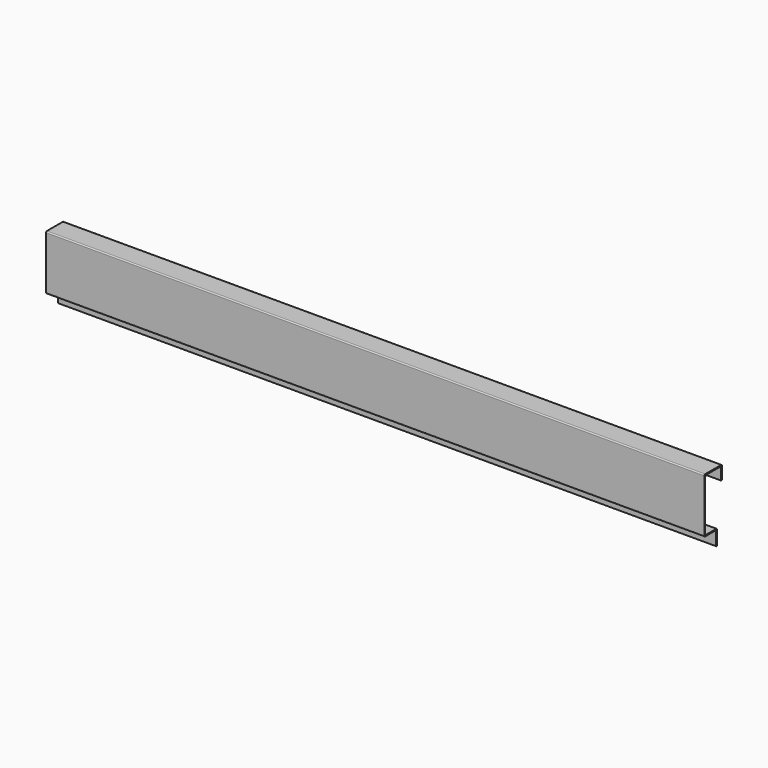
from build123d import *

# Parameters (mm, degrees)
F1_DEPTH = 1200
F3_D     = 5
F4_R     = 2


# Not quite as in the source:
# - a feature names something its author has since deleted; it is built from what else it names


with BuildPart() as f1:
    # F0 (on Right) → F1 (new body)
    with BuildSketch(Plane.YZ):
        Polygon((-18.8378913403, 177.8021101952), (-18.8378913403, 154.8021101952), (-16.8378913403, 154.8021101952), (-16.8378913403, 179.8021101952), (-56.8378913403, 179.8021101952), (-56.8378913403, 79.8021101952), (-29.8378913403, 79.8021101952), (-29.8378913403, 53.8021101952), (-27.8378913403, 53.8021101952), (-27.8378913403, 81.8021101952), (-54.8378913403, 81.8021101952), (-54.8378913403, 177.8021101952), align=None)
    extrude(amount=F1_DEPTH)

    # F3 (through all)
    with Locations(Plane.XZ.offset(29.8378913403)):
        with Locations((433, 66.8021101952), (767, 66.8021101952), (1100, 66.8021101952), (100, 66.8021101952)):
            Hole(F3_D / 2)

    # F4
    f4_edges = [f1.edges().sort_by_distance(p)[0] for p in [
        (600, -56.837891, 179.80211),
        (600, -16.837891, 179.80211),
        (600, -56.837891, 79.80211),
        (600, -27.837891, 81.80211),
        (600, -54.837891, 81.80211),
        (600, -29.837891, 79.80211),
        (600, -18.837891, 177.80211),
        (600, -54.837891, 177.80211),
    ]]
    fillet(f4_edges, radius=F4_R)


solid = f1.part
